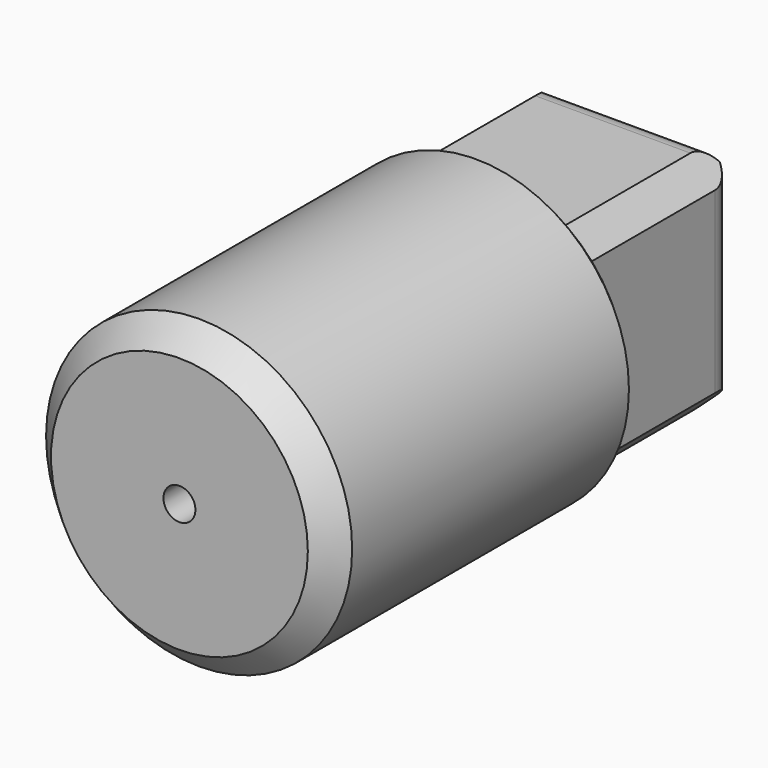
from build123d import *

# Parameters (mm, degrees)
F0_R     = 31.5738283612
F1_DEPTH = 78.994
F3_D     = 6.6
F5_W     = 42.1696881435
F5_H     = 47.0036589152
F5_R     = 3.3
F6_DEPTH = 37.846
F7_SIZE2 = 5.08
F7_SIZE  = 5.08
F8_F1_R  = 5.08
F8_F2_R  = 5.08
F8_F3_R  = 5.0799
F8_F4_R  = 5.0799
F9_SIZE  = 2.54
F10_SIZE = 5.08


# Not quite as in the source:
# - a fillet or chamfer is up to 0.001 mm smaller than in the source, because OpenCascade refuses the exact size


with BuildPart() as f1:
    # F0 (on Front) → F1 (new body)
    with BuildSketch(Plane.XZ):
        Circle(F0_R)
    extrude(amount=F1_DEPTH)

    # F3 (through all)
    with Locations(Plane.XZ.offset(78.994)):
        with Locations((0, 0)):
            Hole(F3_D / 2)

    # F5 (on face) → F6 (join)
    with BuildSketch(Plane(origin=(0, 0, 0), x_dir=(-1, 0, 0), z_dir=(0, 1, 0))):
        Rectangle(F5_W, F5_H)
        Circle(F5_R, mode=Mode.SUBTRACT)
    extrude(amount=F6_DEPTH)

    # F7
    f7_edges = [f1.edges().sort_by_distance(p)[0] for p in [
        (21.084844, 18.923, 23.501829),
        (21.084844, 18.923, -23.501829),
        (-21.084844, 18.923, 23.501829),
        (-21.084844, 18.923, -23.501829),
    ]]
    chamfer(f7_edges, length=F7_SIZE, length2=F7_SIZE2)

    # F8: fillet of radius 5.08 on 4 edges, made by hand

    # F8_f1
    f8_f1_edges = [f1.edges().sort_by_distance(p)[0] for p in [
        (-21.0848440718, 37.846, 0),
    ]]
    fillet(f8_f1_edges, radius=F8_F1_R)

    # F8_f2
    f8_f2_edges = [f1.edges().sort_by_distance(p)[0] for p in [
        (21.0848440718, 37.846, 0),
    ]]
    fillet(f8_f2_edges, radius=F8_F2_R)

    # F8_f3 (radius 5.08 in the source; OpenCascade refuses exactly that, so slightly less here)
    f8_f3_edges = [f1.edges().sort_by_distance(p)[0] for p in [
        (0, 37.846, -23.5018294576),
    ]]
    fillet(f8_f3_edges, radius=F8_F3_R)

    # F8_f4 (radius 5.08 in the source; OpenCascade refuses exactly that, so slightly less here)
    f8_f4_edges = [f1.edges().sort_by_distance(p)[0] for p in [
        (0, 37.846, 23.5018294576),
    ]]
    fillet(f8_f4_edges, radius=F8_F4_R)

    # F9
    f9_edges = [f1.edges().sort_by_distance(p)[0] for p in [
        (-31.573828, 0, 0),
    ]]
    chamfer(f9_edges, length=F9_SIZE)

    # F10
    f10_edges = [f1.edges().sort_by_distance(p)[0] for p in [
        (-31.573828, -78.994, 0),
    ]]
    chamfer(f10_edges, length=F10_SIZE)


solid = f1.part
